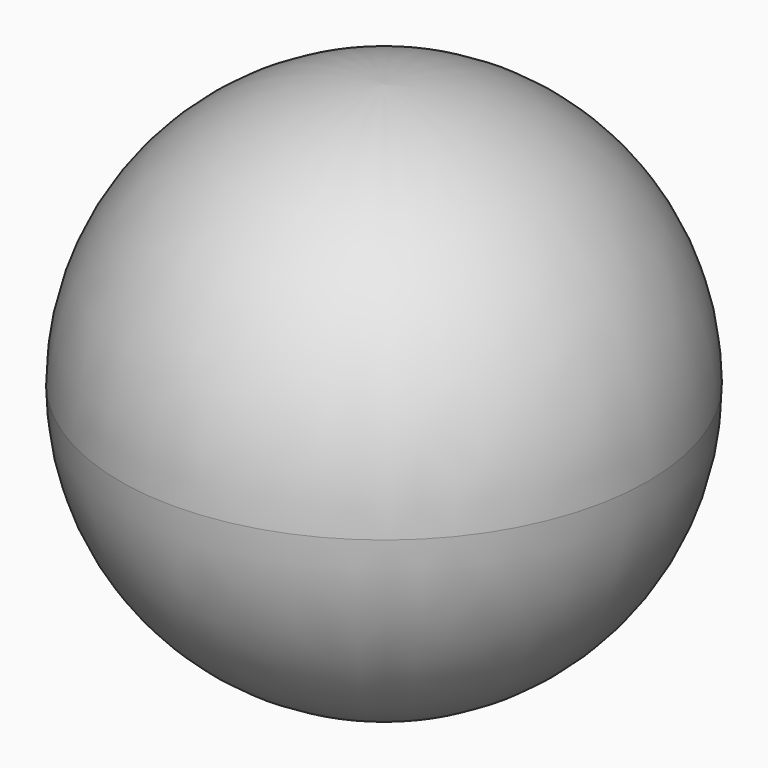
from build123d import *

# Parameters (mm, degrees)
F0_R          = 10.7
F1_DEPTH      = 10.7
F1_DEPTH_BACK = 10.7
F2_R          = 10.69999


# Not quite as in the source:
# - a fillet or chamfer is up to 0.001 mm smaller than in the source, because OpenCascade refuses the exact size


with BuildPart() as f1:
    # F0 (on Top) → F1 (new body, two sides)
    with BuildSketch(Plane.XY) as f1_sk:
        Circle(F0_R)
    extrude(amount=F1_DEPTH)
    extrude(f1_sk.sketch, amount=-F1_DEPTH_BACK)

    # F2 (radius 10.7 in the source; OpenCascade refuses exactly that, so slightly less here)
    f2_edges = [f1.edges().sort_by_distance(p)[0] for p in [
        (10.7, 0, 5.35),
        (-10.7, 0, 0),
        (-10.7, 0, 10.7),
    ]]
    fillet(f2_edges, radius=F2_R)


solid = f1.part
